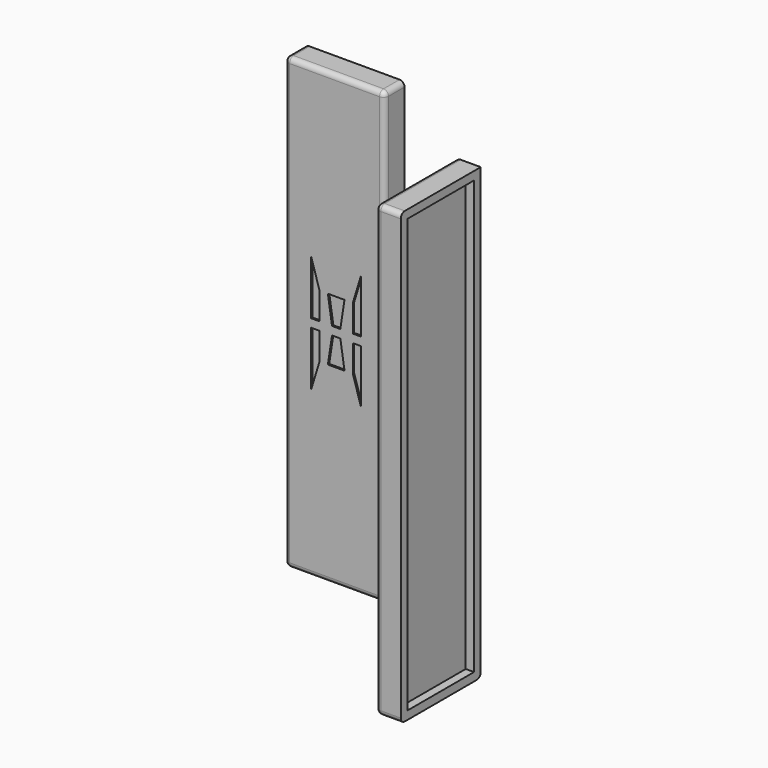
from build123d import *

# Parameters (mm, degrees)
F0_W      = 60
F0_H      = 270
F2_DEPTH  = 15
F3_W      = 50
F3_H      = 260
F4_DEPTH  = 5
F1_W      = 60
F1_H      = 270
F5_DEPTH  = 15
F6_W      = 50
F6_H      = 260
F7_DEPTH  = 5
F9_DEPTH  = 10
F10_R     = 3
F11_R     = 3
F13_DEPTH = 1
F15_DEPTH = 1


# Not quite as in the source:
# - a feature names something its author has since deleted; it is built from what else it names


with BuildPart() as f2:
    # F0 (on Front) → F2 (new body)
    with BuildSketch(Plane.XZ):
        with Locations((-121.8493213905, -25.8904273567)):
            Rectangle(F0_W, F0_H)
    extrude(amount=F2_DEPTH)

    # F3 (on face) → F4 (join)
    with BuildSketch(Plane.XZ):
        with Locations((-121.8493213905, -25.8904273567)):
            Rectangle(F3_W, F3_H)
    extrude(amount=-F4_DEPTH)

    # F8 (on face) → F9 (cut)
    with BuildSketch(Plane(origin=(0, 5, 0), x_dir=(-1, 0, 0), z_dir=(0, 1, 0))):
        with BuildLine():
            Line((109.8493213905, -150.8904273567), (133.8493213905, -150.8904273567))
            Line((133.8493213905, -150.8904273567), (133.8493213905, -45.8904273567))
            add(Edge.make_bspline(
                [(109.8493213905, -45.8904273567), (121.8493213905, -57.1404273567), (133.8493213905, -45.8904273567)],
                knots=[2.4980915448, 2.4980915448, 2.4980915448, 3.7850937624, 3.7850937624, 3.7850937624], degree=2, weights=[1, 0.8, 1]))
            Line((109.8493213905, -45.8904273567), (109.8493213905, -150.8904273567))
        make_face()
        with BuildLine():
            add(Edge.make_bspline(
                [(133.8493213905, -5.8904273567), (128.5159880572, -0.8904273567), (121.8493213905, -0.8904273567)],
                knots=[5.6396841984, 5.6396841984, 5.6396841984, 6.2831853072, 6.2831853072, 6.2831853072], degree=2, weights=[1, 0.9486832981, 1]))
            Line((133.8493213905, -5.8904273567), (133.8493213905, 99.1095726433))
            Line((133.8493213905, 99.1095726433), (109.8493213905, 99.1095726433))
            Line((109.8493213905, 99.1095726433), (109.8493213905, -5.8904273567))
            add(Edge.make_bspline(
                [(121.8493213905, -0.8904273567), (115.1826547239, -0.8904273567), (109.8493213905, -5.8904273567)],
                knots=[0, 0, 0, 0.6435011088, 0.6435011088, 0.6435011088], degree=2, weights=[1, 0.9486832981, 1]))
        make_face()
        with BuildLine():
            Line((133.8493213905, -5.8904273567), (133.8493213905, -45.8904273567))
            add(Edge.make_bspline(
                [(133.8493213905, -45.8904273567), (155.1826547239, -25.8904273567), (133.8493213905, -5.8904273567)],
                knots=[3.7850937624, 3.7850937624, 3.7850937624, 5.6396841984, 5.6396841984, 5.6396841984], degree=2, weights=[1, 0.6, 1]))
        make_face()
        with BuildLine():
            add(Edge.make_bspline(
                [(109.8493213905, -45.8904273567), (121.8493213905, -57.1404273567), (133.8493213905, -45.8904273567)],
                knots=[2.4980915448, 2.4980915448, 2.4980915448, 3.7850937624, 3.7850937624, 3.7850937624], degree=2, weights=[1, 0.8, 1]))
            Line((133.8493213905, -45.8904273567), (133.8493213905, -5.8904273567))
            add(Edge.make_bspline(
                [(133.8493213905, -5.8904273567), (128.5159880572, -0.8904273567), (121.8493213905, -0.8904273567)],
                knots=[5.6396841984, 5.6396841984, 5.6396841984, 6.2831853072, 6.2831853072, 6.2831853072], degree=2, weights=[1, 0.9486832981, 1]))
            add(Edge.make_bspline(
                [(121.8493213905, -0.8904273567), (115.1826547239, -0.8904273567), (109.8493213905, -5.8904273567)],
                knots=[0, 0, 0, 0.6435011088, 0.6435011088, 0.6435011088], degree=2, weights=[1, 0.9486832981, 1]))
            Line((109.8493213905, -5.8904273567), (109.8493213905, -45.8904273567))
        make_face()
        with BuildLine():
            add(Edge.make_bspline(
                [(109.8493213905, -5.8904273567), (88.5159880572, -25.8904273567), (109.8493213905, -45.8904273567)],
                knots=[0.6435011088, 0.6435011088, 0.6435011088, 2.4980915448, 2.4980915448, 2.4980915448], degree=2, weights=[1, 0.6, 1]))
            Line((109.8493213905, -45.8904273567), (109.8493213905, -5.8904273567))
        make_face()
    extrude(amount=-F9_DEPTH, mode=Mode.SUBTRACT)

    # F10
    f10_edges = [f2.edges().sort_by_distance(p)[0] for p in [
        (-121.849321, -15, 109.109573),
        (-151.849321, -7.5, 109.109573),
        (-91.849321, -7.5, 109.109573),
        (-91.849321, -15, -25.890427),
        (-151.849321, -15, -25.890427),
        (-121.849321, -15, -160.890427),
        (-151.849321, -7.5, -160.890427),
        (-91.849321, -7.5, -160.890427),
    ]]
    fillet(f10_edges, radius=F10_R)

    # F14 (on face) → F15 (cut)
    with BuildSketch(Plane.XZ.offset(15)):
        Polygon((-135.9017485874, 8.1252877414), (-135.9017485874, -24.3747122586), (-130.9017485874, -24.3747122586), (-130.9017485874, -8.1227890678), align=None)
        Polygon((-120.9017493272, -8.1208656498), (-125.9017493272, -8.1208658774), (-123.4017485874, -24.3747122586), (-118.4017485874, -24.3747122586), (-115.9017493272, -8.1208654223), align=None)
        Polygon((-105.9080004363, 8.1349024923), (-110.9017504368, -8.1150963056), (-110.8954993276, -24.3670182942), (-105.8954996975, -24.3650951036), align=None)
        Polygon((-130.9017485874, -29.3747122586), (-135.9017485874, -29.3747122586), (-135.9017485874, -45.6247122586), (-135.9017485874, -61.8747122586), (-130.9017485874, -45.6247122586), align=None)
        Polygon((-105.8998287257, -29.3843281183), (-110.8998283559, -29.3824049277), (-110.8998283559, -45.6324049277), (-105.8998287257, -61.8843281183), align=None)
        Polygon((-123.4017485874, -29.3747122586), (-125.9002702644, -45.6189424591), (-115.903228459, -45.6189424591), (-118.4017485874, -29.3747122586), align=None)
    extrude(amount=-F15_DEPTH, mode=Mode.SUBTRACT)


with BuildPart() as f5:
    # F1 (on Right) → F5 (new body)
    with BuildSketch(Plane.YZ):
        with Locations((-106.3447256267, -5.4207965732)):
            Rectangle(F1_W, F1_H)
    extrude(amount=F5_DEPTH)

    # F6 (on face) → F7 (cut)
    with BuildSketch(Plane.YZ.offset(15)):
        with Locations((-106.3447256267, -5.4207965732)):
            Rectangle(F6_W, F6_H)
    extrude(amount=-F7_DEPTH, mode=Mode.SUBTRACT)

    # F11
    f11_edges = [f5.edges().sort_by_distance(p)[0] for p in [
        (7.5, -136.344726, 129.579203),
        (0, -106.344726, 129.579203),
        (0, -136.344726, -5.420797),
        (0, -76.344726, -5.420797),
        (0, -106.344726, -140.420797),
        (7.5, -76.344726, -140.420797),
        (7.5, -136.344726, -140.420797),
    ]]
    fillet(f11_edges, radius=F11_R)

    # F12 (on face) → F13 (cut)
    with BuildSketch(Plane(origin=(0, 0, 0), x_dir=(0, -1, 0), z_dir=(-1, 0, 0))):
        Polygon((105.4581373974, -56.0113014256), (95.4581373974, -56.0113014256), (99.5036673885, -70.4574153882), (101.4126074063, -70.4574153882), align=None)
        Polygon((90.9570677645, -70.4574153882), (90.9570677645, -39.9385087348), (86.4559981315, -23.8657160441), (86.4559981315, -70.4574153882), align=None)
        Polygon((114.4602766633, -23.8657160441), (109.9592070304, -39.9385087348), (109.9592070304, -70.4574153882), (114.4602766633, -70.4574153882), align=None)
        Polygon((109.9592070304, -77.2740167), (109.9592070304, -107.7929233534), (114.4602766633, -123.8657160441), (114.4602766633, -77.2740167), align=None)
        Polygon((99.5036673885, -77.2740167), (95.4581373974, -91.7201306627), (105.4581373974, -91.7201306627), (101.4126074063, -77.2740167), align=None)
        Polygon((86.4559981315, -123.8657160441), (90.9570677645, -107.7929233534), (90.9570677645, -77.2740167), (86.4559981315, -77.2740167), align=None)
    extrude(amount=-F13_DEPTH, mode=Mode.SUBTRACT)


solid = Compound([f2.part, f5.part])
